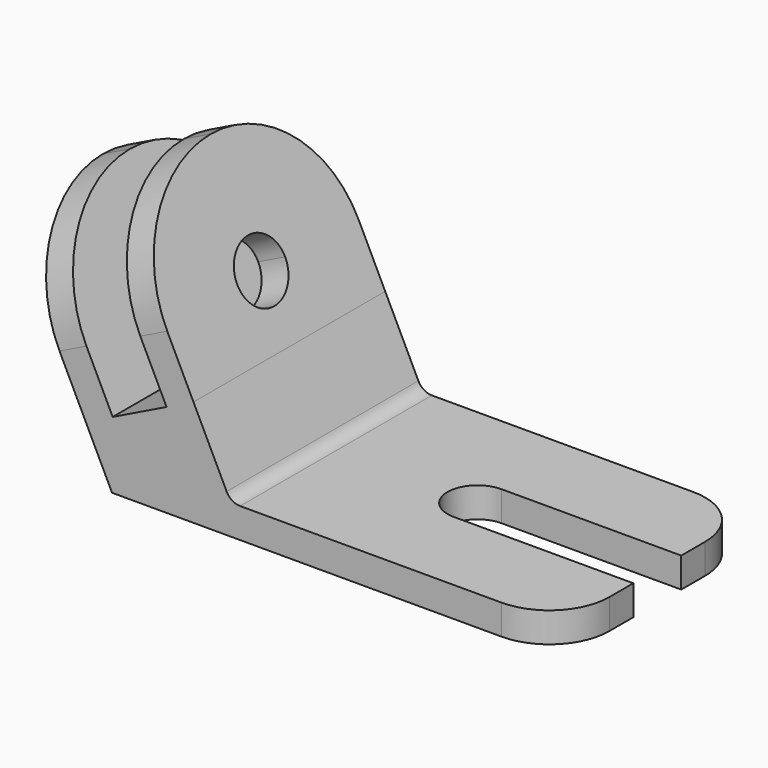
from build123d import *

# Parameters (mm, degrees)
F1_DEPTH      = 40
F1_DEPTH_BACK = 40
F2_R          = 39.99999
F4_DEPTH      = 25
F5_R          = 20
F6_R          = 5
F8_DEPTH      = 63


# Not quite as in the source:
# - a fillet or chamfer is up to 0.001 mm smaller than in the source, because OpenCascade refuses the exact size


with BuildPart() as f1:
    # F0 (on Front) → F1 (new body, two sides)
    with BuildSketch(Plane.XZ) as f1_sk:
        Polygon((-75, 0), (0, 0), (75, 0), (75, 10), (-35.3732482667, 10), (-47.8156610838, 35.5107267975), (-74.1179298912, 89.4383695755), (-83.1058703542, 85.0546581076), (-56.8036015468, 31.1270153297), (-74.7794824728, 22.3595923939), (-101.0817512801, 76.2872351718), (-110.0696917431, 71.9035237039), align=None)
    extrude(amount=F1_DEPTH)
    extrude(f1_sk.sketch, amount=-F1_DEPTH_BACK)

    # F2 (radius 40 in the source; OpenCascade refuses exactly that, so slightly less here)
    f2_edges = [f1.edges().sort_by_distance(p)[0] for p in [
        (-78.6119, -40, 87.246514),
        (-78.6119, 40, 87.246514),
        (-105.575722, -40, 74.095379),
        (-105.575722, 40, 74.095379),
    ]]
    fillet(f2_edges, radius=F2_R)

    # F3 (on face) → F4 (cut)
    with BuildSketch(Plane.XY.offset(10)):
        with BuildLine():
            Line((75, 10), (15, 10))
            ThreePointArc((15, 10), (5, 0), (15, -10))
            Line((15, -10), (75, -10))
            Line((75, -10), (75, 10))
        make_face()
    extrude(amount=-F4_DEPTH, mode=Mode.SUBTRACT)

    # F5
    f5_edges = [f1.edges().sort_by_distance(p)[0] for p in [
        (75, 40, 5),
        (75, -40, 5),
    ]]
    fillet(f5_edges, radius=F5_R)

    # F6
    f6_edges = [f1.edges().sort_by_distance(p)[0] for p in [
        (-35.373248, 0, 10),
    ]]
    fillet(f6_edges, radius=F6_R)

    # F7 (on face) → F8 (cut)
    with BuildSketch(Plane(origin=(-24.6355434727, 0, -12.0155573887), x_dir=(0, 1, 0), z_dir=(0.8987940463, 0, 0.4383711468))):
        with BuildLine():
            ThreePointArc((0, 64.3188986308), (7.0710678119, 67.247830819), (10, 74.3188986308))
            ThreePointArc((10, 74.3188986308), (-7.0710678119, 81.3899664427), (0, 64.3188986308))
        make_face()
    extrude(amount=-F8_DEPTH, mode=Mode.SUBTRACT)


solid = f1.part
